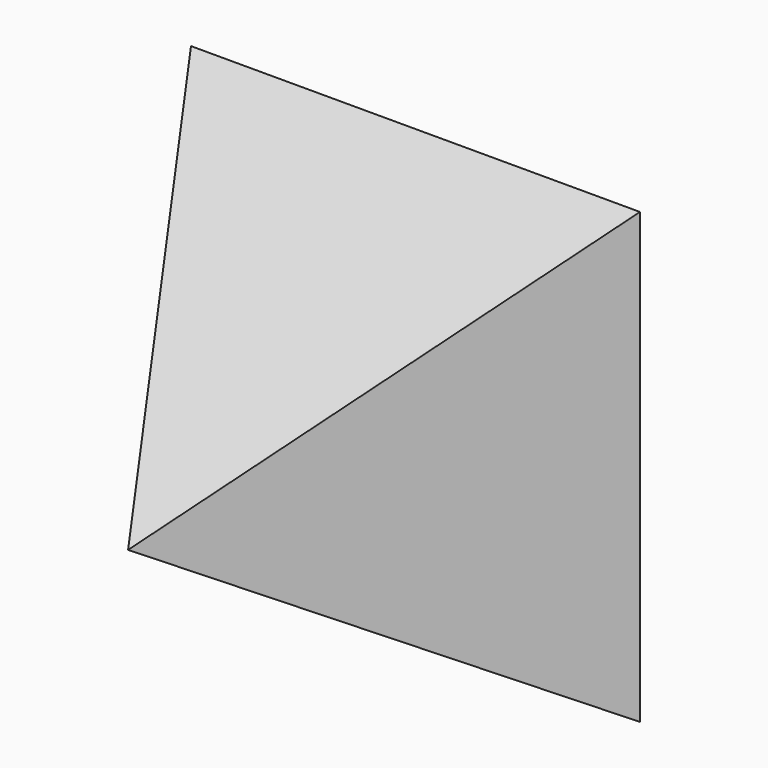
from build123d import *

# Parameters (mm, degrees)
F0_W = 152.4
F0_H = 152.4


# Not quite as in the source:
# - an extrude whose draft closes it to a point is written as a loft to that point


with BuildPart() as f1:
    # F0 (on Front) → F1 section 0
    with BuildSketch(Plane.XZ, mode=Mode.PRIVATE) as f1_s0:
        with Locations((1.8629767001, -9.8051466048)):
            Rectangle(F0_W, F0_H)
    loft([f1_s0.sketch, Vertex(1.8629767001, -121.9454911129, -9.8051466048)], ruled=True)


solid = f1.part
